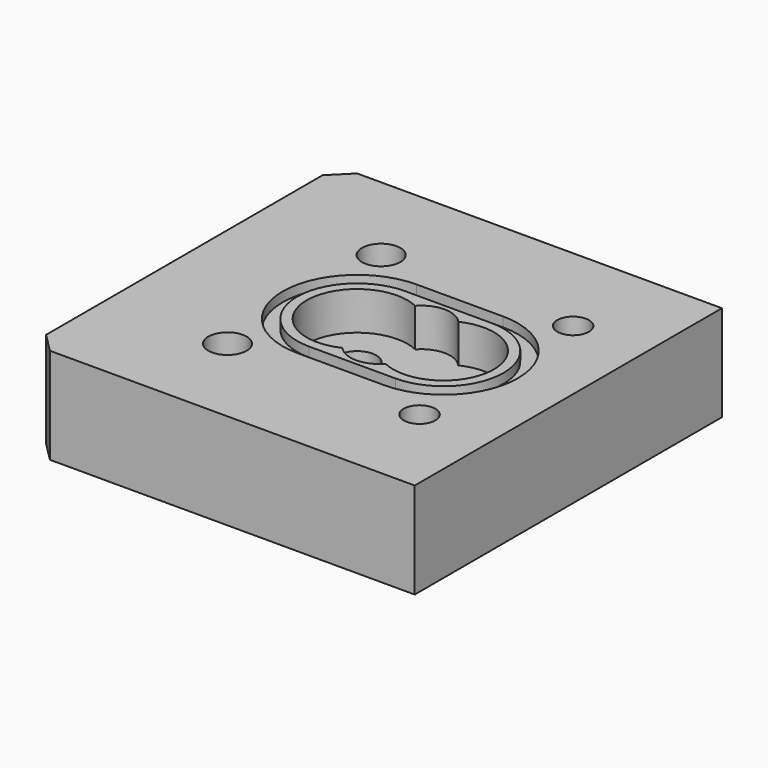
from build123d import *

# Parameters (mm, degrees)
F0_W      = 41
F0_H      = 40
F0_R      = 2
F0_R_2    = 1.65
F1_DEPTH  = 10
F2_DEPTH  = 1
F3_DEPTH  = 8
F4_DEPTH  = 4
F5_R      = 4
F5_R_2    = 2
F6_DEPTH  = 1
F7_DEPTH  = 8
F8_DEPTH  = 2
F9_SIZE   = 2
F10_DEPTH = 3


# Not quite as in the source:
# - a feature names something its author has since deleted; it is built from what else it names


with BuildPart() as f1:
    # F0 (on Top) → F1 (new body)
    with BuildSketch(Plane.XY):
        with Locations((20.5, -20)):
            Rectangle(F0_W, F0_H)
        with Locations((10.5, -30)):
            Circle(F0_R, mode=Mode.SUBTRACT)
        with Locations((30.5, -30)):
            Circle(F0_R_2, mode=Mode.SUBTRACT)
        with Locations((10.5, -10)):
            Circle(F0_R, mode=Mode.SUBTRACT)
        with BuildLine():
            Line((25, -27.75), (16, -27.75))
            ThreePointArc((16, -27.75), (8.25, -20), (16, -12.25))
            Line((16, -12.25), (25, -12.25))
            ThreePointArc((25, -12.25), (32.75, -20), (25, -27.75))
        make_face(mode=Mode.SUBTRACT)
        with Locations((30.5, -10)):
            Circle(F0_R_2, mode=Mode.SUBTRACT)
        with BuildLine():
            ThreePointArc((16, -12.25), (8.25, -20), (16, -27.75))
            Line((16, -27.75), (25, -27.75))
            ThreePointArc((25, -27.75), (32.75, -20), (25, -12.25))
            Line((25, -12.25), (16, -12.25))
        make_face()
        with BuildLine():
            ThreePointArc((16, -26.25), (9.75, -20), (16, -13.75))
            Line((16, -13.75), (25, -13.75))
            ThreePointArc((25, -13.75), (31.25, -20), (25, -26.25))
            Line((25, -26.25), (16, -26.25))
        make_face(mode=Mode.SUBTRACT)
        with BuildLine():
            Line((25, -13.75), (16, -13.75))
            ThreePointArc((16, -13.75), (9.75, -20), (16, -26.25))
            Line((16, -26.25), (25, -26.25))
            ThreePointArc((25, -26.25), (31.25, -20), (25, -13.75))
        make_face()
        with BuildLine():
            ThreePointArc((22.7443308628, -15.25927677), (30.25, -20), (22.7443308628, -24.74072323))
            ThreePointArc((22.7443308628, -24.74072323), (20.5, -25.75), (18.2556691372, -24.74072323))
            ThreePointArc((18.2556691372, -24.74072323), (10.75, -20), (18.2556691372, -15.25927677))
            ThreePointArc((18.2556691372, -15.25927677), (20.5, -14.25), (22.7443308628, -15.25927677))
        make_face(mode=Mode.SUBTRACT)
        with BuildLine():
            ThreePointArc((18.2556691372, -24.74072323), (20.5, -25.75), (22.7443308628, -24.74072323))
            ThreePointArc((22.7443308628, -24.74072323), (30.25, -20), (22.7443308628, -15.25927677))
            ThreePointArc((22.7443308628, -15.25927677), (20.5, -14.25), (18.2556691372, -15.25927677))
            ThreePointArc((18.2556691372, -15.25927677), (10.75, -20), (18.2556691372, -24.74072323))
        make_face()
        with Locations((16, -20)):
            Circle(F0_R, mode=Mode.SUBTRACT)
        with Locations((25, -20)):
            Circle(F0_R, mode=Mode.SUBTRACT)
        with Locations((25, -20)):
            Circle(F0_R)
        with Locations((30.5, -10)):
            Circle(F0_R_2)
        with Locations((30.5, -30)):
            Circle(F0_R_2)
    extrude(amount=-F1_DEPTH)

    # F0 (on Top) → F2 (cut)
    with BuildSketch(Plane.XY):
        with BuildLine():
            ThreePointArc((16, -12.25), (8.25, -20), (16, -27.75))
            Line((16, -27.75), (25, -27.75))
            ThreePointArc((25, -27.75), (32.75, -20), (25, -12.25))
            Line((25, -12.25), (16, -12.25))
        make_face()
        with BuildLine():
            ThreePointArc((16, -26.25), (9.75, -20), (16, -13.75))
            Line((16, -13.75), (25, -13.75))
            ThreePointArc((25, -13.75), (31.25, -20), (25, -26.25))
            Line((25, -26.25), (16, -26.25))
        make_face(mode=Mode.SUBTRACT)
    extrude(amount=-F2_DEPTH, mode=Mode.SUBTRACT)

    # F0 (on Top) → F3 (cut)
    with BuildSketch(Plane.XY):
        with Locations((25, -20)):
            Circle(F0_R)
    extrude(amount=-F3_DEPTH, mode=Mode.SUBTRACT)

    # F0 (on Top) → F4 (cut)
    with BuildSketch(Plane.XY):
        with BuildLine():
            ThreePointArc((18.2556691372, -24.74072323), (20.5, -25.75), (22.7443308628, -24.74072323))
            ThreePointArc((22.7443308628, -24.74072323), (30.25, -20), (22.7443308628, -15.25927677))
            ThreePointArc((22.7443308628, -15.25927677), (20.5, -14.25), (18.2556691372, -15.25927677))
            ThreePointArc((18.2556691372, -15.25927677), (10.75, -20), (18.2556691372, -24.74072323))
        make_face()
        with Locations((16, -20)):
            Circle(F0_R, mode=Mode.SUBTRACT)
        with Locations((25, -20)):
            Circle(F0_R, mode=Mode.SUBTRACT)
    extrude(amount=-F4_DEPTH, mode=Mode.SUBTRACT)

    # F5 (on face) → F6 (cut)
    with BuildSketch(Plane(origin=(0, 0, -10), x_dir=(1, 0, 0), z_dir=(0, 0, -1))):
        with Locations((16, 20)):
            Circle(F5_R)
        with Locations((16, 20)):
            Circle(F5_R_2, mode=Mode.SUBTRACT)
    extrude(amount=-F6_DEPTH, mode=Mode.SUBTRACT)

    # F0 (on Top) → F7 (cut)
    with BuildSketch(Plane.XY):
        with Locations((30.5, -30)):
            Circle(F0_R_2)
        with Locations((30.5, -10)):
            Circle(F0_R_2)
    extrude(amount=-F7_DEPTH, mode=Mode.SUBTRACT)

    # F8 (add): a face of the model
    f8_faces = [f1.faces().sort_by_distance(p)[0] for p in [
        (0, -20, -5),
    ]]
    extrude(f8_faces, amount=F8_DEPTH)

    # F9
    f9_edges = [f1.edges().sort_by_distance(p)[0] for p in [
        (-2, -40, -5),
        (-2, 0, -5),
    ]]
    chamfer(f9_edges, length=F9_SIZE)

    # F10 (cut): a face of the model
    f10_faces = [f1.faces().sort_by_distance(p)[0] for p in [
        (41, -20, -5),
    ]]
    extrude(f10_faces, amount=-F10_DEPTH, mode=Mode.SUBTRACT)


solid = f1.part
